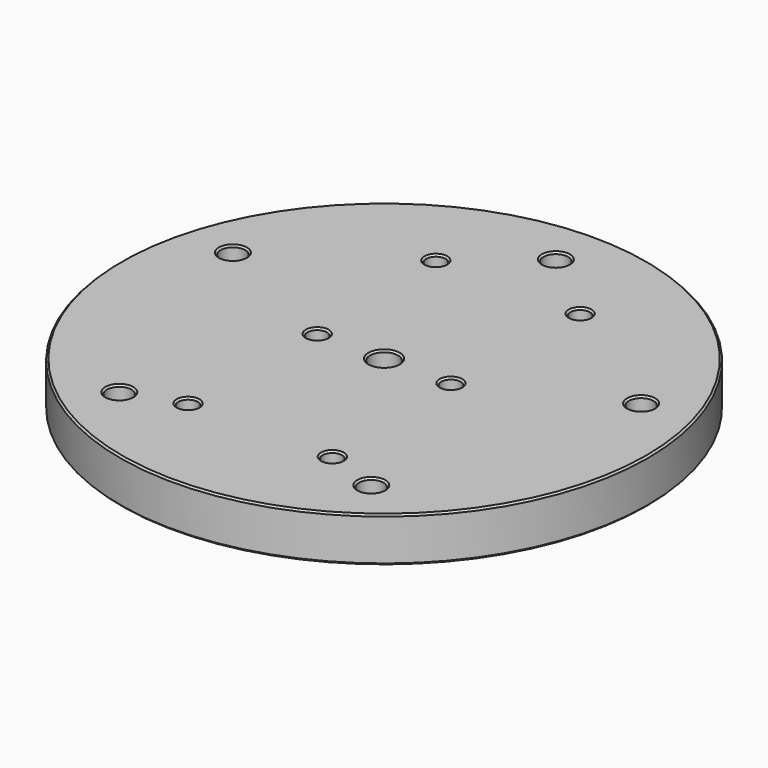
from build123d import *

# Parameters (mm, degrees)
F0_R           = 75
F1_DEPTH       = 12.7
F2_D           = 5.5
F2_CBORE_D     = 9.75
F2_CBORE_DEPTH = 5
F4_D           = 7
F5_D           = 7.9375
F6_SIZE        = 0.5


# Not quite as in the source:
# - a length typed as a fraction of an inch, garbled in the dataset ("3 / 203.2 mm" for 3/8 in), is restored


with BuildPart() as f1:
    # F0 (on Top) → F1 (new body)
    with BuildSketch(Plane.XY):
        Circle(F0_R)
    extrude(amount=F1_DEPTH)

    # F2 (through all)
    with Locations(Plane(origin=(0, 0, 0), x_dir=(1, 0, 0), z_dir=(0, 0, -1))):
        with Locations((-20.5, -44), (20.5, -44), (-19, 0), (19, 0), (-20.5, 44), (20.5, 44)):
            CounterBoreHole(F2_D / 2, F2_CBORE_D / 2, F2_CBORE_DEPTH)

    # F4 (through all)
    with Locations(Plane.XY.offset(12.7)):
        with Locations((0, 61), (58, 18.8), (-58, 18.8), (-35.8, -49.3), (35.8, -49.3)):
            Hole(F4_D / 2)

    # F5 (through all)
    with Locations(Plane(origin=(0, 0, 0), x_dir=(1, 0, 0), z_dir=(0, 0, -1))):
        with Locations((0, 0)):
            Hole(F5_D / 2)

    # F6
    f6_edges = [f1.edges().sort_by_distance(p)[0] for p in [
        (-75, 0, 0),
        (-39.3, -49.3, 0),
        (-25.375, -44, 0),
        (-23.875, 0, 0),
        (15.625, -44, 0),
        (32.3, -49.3, 0),
        (-3.96875, 0, 0),
        (14.125, 0, 0),
        (-61.5, 18.8, 0),
        (-25.375, 44, 0),
        (54.5, 18.8, 0),
        (15.625, 44, 0),
        (-3.5, 61, 0),
        (-75, 0, 12.7),
        (-39.3, -49.3, 12.7),
        (-23.25, -44, 12.7),
        (-21.75, 0, 12.7),
        (17.75, -44, 12.7),
        (32.3, -49.3, 12.7),
        (-3.96875, 0, 12.7),
        (16.25, 0, 12.7),
        (-61.5, 18.8, 12.7),
        (-23.25, 44, 12.7),
        (54.5, 18.8, 12.7),
        (17.75, 44, 12.7),
        (-3.5, 61, 12.7),
    ]]
    chamfer(f6_edges, length=F6_SIZE)


solid = f1.part
